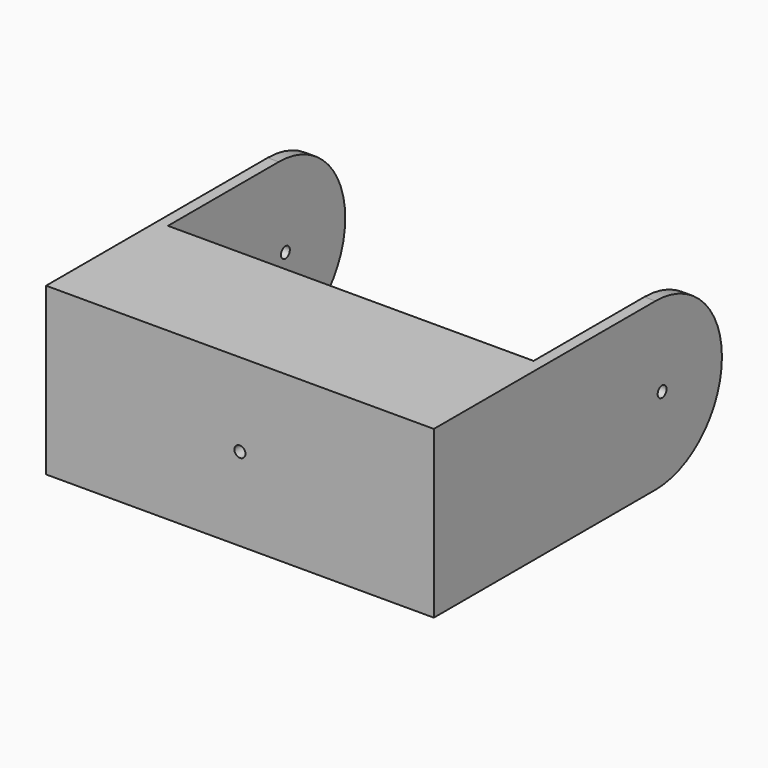
from build123d import *

# Parameters (mm, degrees)
F0_W     = 2
F0_H     = 30
F0_W_2   = 66
F0_R     = 1
F1_DEPTH = 25
F2_DEPTH = 25
F3_R     = 1
F4_DEPTH = 2
F5_R     = 1
F6_DEPTH = 2


# Not quite as in the source:
# - a feature names something its author has since deleted; it is built from what else it names


with BuildPart() as f1:
    # F0 (on Front) → F1 (new body)
    with BuildSketch(Plane.XZ):
        with Locations((-34, 0)):
            Rectangle(F0_W, F0_H)
        with Locations((34, 0)):
            Rectangle(F0_W, F0_H)
        Rectangle(F0_W_2, F0_H)
        Circle(F0_R, mode=Mode.SUBTRACT)
    extrude(amount=F1_DEPTH)

    # F0 (on Front) → F2 (join)
    with BuildSketch(Plane.XZ):
        with Locations((34, 0)):
            Rectangle(F0_W, F0_H)
        with Locations((-34, 0)):
            Rectangle(F0_W, F0_H)
    extrude(amount=-F2_DEPTH)

    # F3 (on face) → F4 (join)
    with BuildSketch(Plane.YZ.offset(35)):
        with BuildLine():
            Line((25, 15), (25, -15))
            ThreePointArc((25, -15), (40, 0), (25, 15))
        make_face()
        with Locations((26.5, 0)):
            Circle(F3_R, mode=Mode.SUBTRACT)
    extrude(amount=-F4_DEPTH)

    # F5 (on face) → F6 (join)
    with BuildSketch(Plane(origin=(-35, 0, 0), x_dir=(0, -1, 0), z_dir=(-1, 0, 0))):
        with BuildLine():
            Line((-25, -15), (-25, 15))
            ThreePointArc((-25, 15), (-40, 0), (-25, -15))
        make_face()
        with Locations((-26.5, 0)):
            Circle(F5_R, mode=Mode.SUBTRACT)
    extrude(amount=-F6_DEPTH)


solid = f1.part
